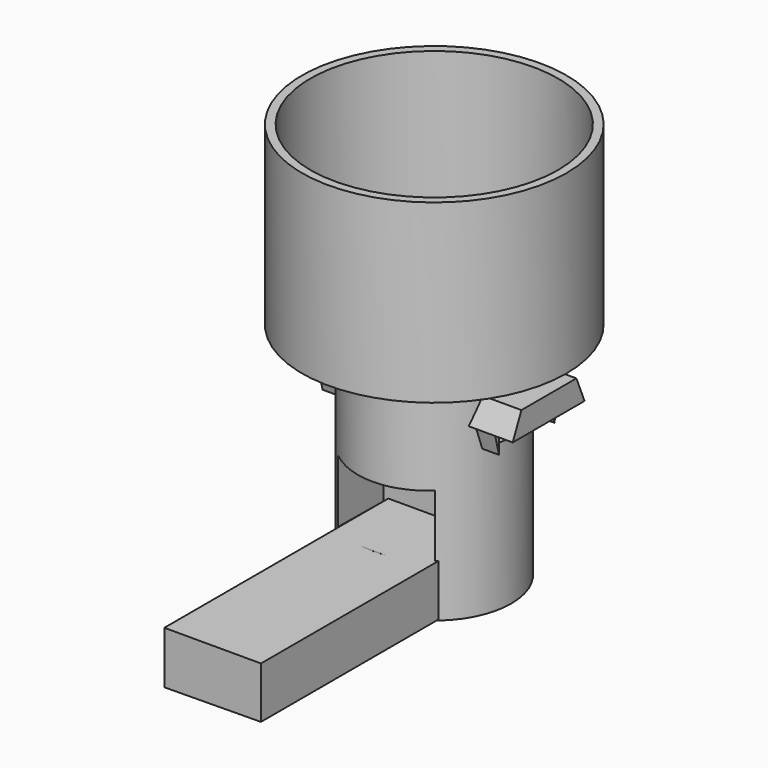
from build123d import *

# Parameters (mm, degrees)
F0_R           = 152.4
F1_DEPTH       = 203.2
F2_R           = 88.9
F3_DEPTH       = 254
F4_W           = 118.0947571993
F4_H           = 79.6899646521
F5_DEPTH       = 152.4
F5_TAPER       = 3
F6_W           = 94.8493182659
F6_H           = 110.4671433568
F7_DEPTH       = 325.12
F8_R           = 142.764871417
F9_DEPTH       = 152.4
F10_W          = 79.6899646521
F10_H          = 52.806597203
F11_DEPTH      = 101.6
F11_DEPTH_BACK = 101.6
F13_DEPTH      = 127
F13_DEPTH_BACK = 127
F15_DEPTH      = 101.6
F15_DEPTH_BACK = 101.6
F17_DEPTH      = 322.505


with BuildPart() as f1:
    # F0 (on Top) → F1 (new body)
    with BuildSketch(Plane.XY):
        Circle(F0_R)
    extrude(amount=F1_DEPTH)

    # F2 (on face) → F3 (join)
    with BuildSketch(Plane(origin=(0, 0, 0), x_dir=(1, 0, 0), z_dir=(0, 0, -1))):
        Circle(F2_R)
    extrude(amount=F3_DEPTH)

    # F4 (on Front) → F5 (cut)
    with BuildSketch(Plane.XZ):
        with Locations((0.4800595343, -158.3820804954)):
            Rectangle(F4_W, F4_H)
    extrude(amount=F5_DEPTH, taper=F5_TAPER, mode=Mode.SUBTRACT)

    # F6 (on face) → F7 (cut)
    with BuildSketch(Plane.XY.offset(203.2)):
        Rectangle(F6_W, F6_H)
    extrude(amount=-F7_DEPTH, mode=Mode.SUBTRACT)

    # F8 (on face) → F9 (cut)
    with BuildSketch(Plane.XY.offset(203.2)):
        Circle(F8_R)
    extrude(amount=-F9_DEPTH, mode=Mode.SUBTRACT)

    # F10 (on Right) → F11 (cut, two sides)
    with BuildSketch(Plane.YZ) as f11_sk:
        with Locations((6.1672367156, -58.5296023637)):
            Rectangle(F10_W, F10_H)
    extrude(amount=F11_DEPTH, mode=Mode.SUBTRACT)
    extrude(f11_sk.sketch, amount=-F11_DEPTH_BACK, mode=Mode.SUBTRACT)

    # F12 (on Right) → F13 (join, two sides)
    with BuildSketch(Plane.YZ) as f13_sk:
        Polygon((45.9540584598, -31.9147333503), (-33.2359305319, -31.9147333503), (-45.800998807, -59.6464499831), (57.6868057251, -59.6464499831), align=None)
    extrude(amount=F13_DEPTH)
    extrude(f13_sk.sketch, amount=-F13_DEPTH_BACK)

    # F14 (on Right) → F15 (join, two sides)
    with BuildSketch(Plane.YZ) as f15_sk:
        Polygon((-33.7745137513, -59.7862656422), (-40.2827188373, -59.6054829657), (-33.7745137513, -85.3911563754), align=None)
        Polygon((53.6378957331, -59.6221797168), (45.722966075, -59.6221797168), (45.800998807, -85.1639956236), align=None)
    extrude(amount=F15_DEPTH)
    extrude(f15_sk.sketch, amount=-F15_DEPTH_BACK)

    # F16 (on Front) → F17 (join)
    with BuildSketch(Plane.XZ):
        Polygon((58.3297610283, -193.6283260584), (-52.9678873718, -193.6283260584), (-52.9678873718, -254.0221810341), (58.3297610283, -252.9366910458), align=None)
    extrude(amount=F17_DEPTH)


solid = f1.part
